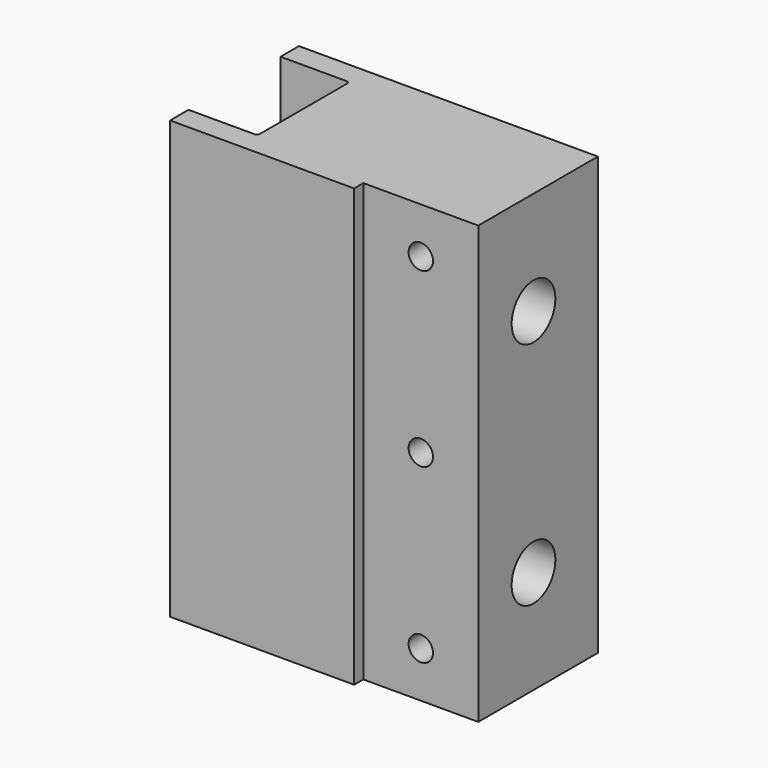
from build123d import *

# Parameters (mm, degrees)
F1_DEPTH       = 120.65
F2_R           = 1.524
F4_D           = 20.6375
F4_CBORE_D     = 30.1752
F4_CBORE_DEPTH = 28.448
F5_W           = 63.5
F5_H           = 241.3
F6_DEPTH       = 6.35
F8_D           = 13.49248
F8_DEPTH       = 41.2172727273
F8_TIP         = 4.0535499425


# Not quite as in the source:
# - a length typed as a fraction of an inch, garbled in the dataset ("3 / 203.2 mm" for 3/8 in), is restored


with BuildPart() as f1:
    # F0 (on Top) → F1 (new body, symmetric)
    with BuildSketch(Plane.XY):
        Polygon((82.55, 44.45), (-82.55, 44.45), (-82.55, 31.75), (-44.45, 31.75), (-44.45, -31.75), (-82.55, -31.75), (-82.55, -44.45), (82.55, -44.45), align=None)
    extrude(amount=F1_DEPTH, both=True)

    # F2
    f2_edges = [f1.edges().sort_by_distance(p)[0] for p in [
        (-44.45, 31.75, 0),
        (-44.45, -31.75, 0),
    ]]
    fillet(f2_edges, radius=F2_R)

    # F4 (through all)
    with Locations(Plane.YZ.offset(82.55)):
        with Locations((0, 63.5), (0, -63.5)):
            CounterBoreHole(F4_D / 2, F4_CBORE_D / 2, F4_CBORE_DEPTH)

    # F5 (on face) → F6 (cut)
    with BuildSketch(Plane.XZ.offset(44.45)):
        with Locations((50.8, 0)):
            Rectangle(F5_W, F5_H)
    extrude(amount=-F6_DEPTH, mode=Mode.SUBTRACT)

    # F8
    with Locations(Plane.XZ.offset(38.1)):
        with Locations((50.8, 95.25), (50.8, 0), (50.8, -95.25)):
            Hole(F8_D / 2, depth=F8_DEPTH)
            with Locations((0, 0, -(F8_DEPTH + F8_TIP / 2))):  # 118° drill point
                Cone(0, F8_D / 2, F8_TIP, mode=Mode.SUBTRACT)


solid = f1.part
